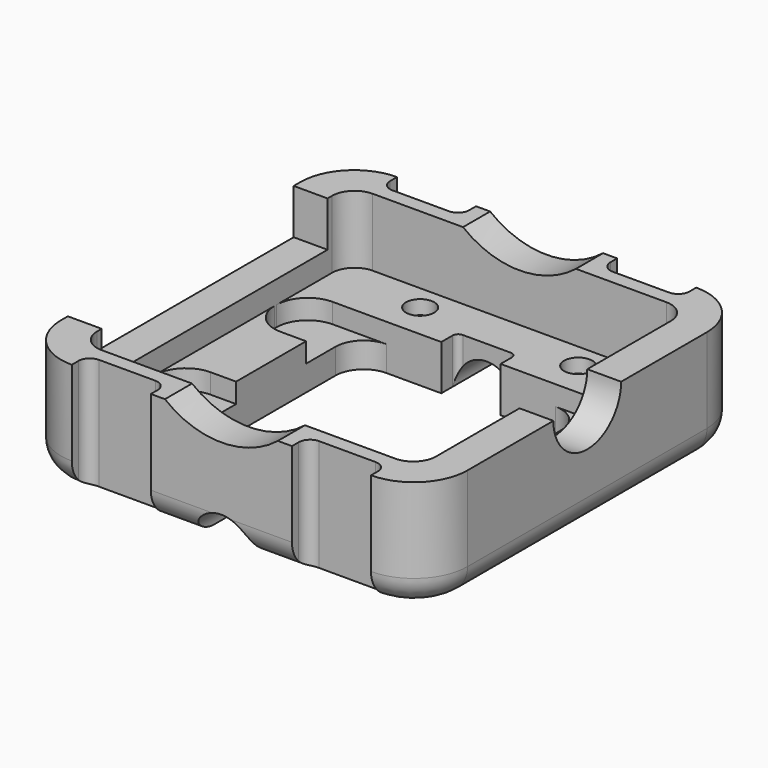
from build123d import *

# Parameters (mm, degrees)
F0_W           = 72
F0_H           = 72
F1_DEPTH       = 20
F2_W           = 60
F2_H           = 59.9999963053
F3_DEPTH       = 12
F4_W           = 40
F4_H           = 38.5
F5_DEPTH       = 8
F6_R           = 5.25
F7_DEPTH       = 72
F8_W           = 50
F8_H           = 16
F9_DEPTH       = 6.5
F10_R          = 7.5
F11_DEPTH      = 6.5
F12_W          = 10.5
F12_H          = 45.5
F13_DEPTH      = 12.001
F13_DEPTH_BACK = 8.001
F14_W          = 60
F14_H          = 11.5
F15_DEPTH      = 3.5
F16_W          = 14
F16_H          = 7
F17_DEPTH      = 20.001
F19_DEPTH      = 72.001
F21_T1_DEPTH   = 4.5
F21_T3_DEPTH   = 97
F21_T5_DEPTH   = 34.5
F21_T7_DEPTH   = 32.25
F21_T9_DEPTH   = 34.5
F21_T11_DEPTH  = 32.25
F22_R          = 2
F23_R          = 5.5
F24_R          = 4
F25_T4_DEPTH   = 8
F25_S5_R       = 5.25
F25_T6_DEPTH   = 6
F25_T10_DEPTH  = 8
F25_S11_R      = 5.25
F25_T12_DEPTH  = 6
F25_T16_DEPTH  = 8
F25_S17_R      = 5.25
F25_T18_DEPTH  = 6
F25_T22_DEPTH  = 8
F25_S23_R      = 5.25
F25_T24_DEPTH  = 6
F20_R          = 4.75
F20_R_2        = 2.5
F26_DEPTH      = 5.5
F27_DEPTH      = 20.0010001
F28_T1_DEPTH   = 43.7500000001
F28_T4_ANGLE   = 90
F28_T6_ANGLE   = 90
F28_T8_ANGLE   = 90
F28_T10_ANGLE  = 90


# Not quite as in the source:
# - a fillet or chamfer that OpenCascade refuses, or shapes differently, is made with other operations: its cross-section is extruded or revolved along the edge and cut away or added


with BuildPart() as f1:
    # F0 (on Top) → F1 (new body)
    with BuildSketch(Plane.XY):
        Rectangle(F0_W, F0_H)
    extrude(amount=F1_DEPTH)

    # F2 (on face) → F3 (cut)
    with BuildSketch(Plane.XY.offset(20)):
        Rectangle(F2_W, F2_H)
    extrude(amount=-F3_DEPTH, mode=Mode.SUBTRACT)

    # F4 (on face) → F5 (cut, through all)
    with BuildSketch(Plane.XY.offset(8)):
        Rectangle(F4_W, F4_H)
    extrude(amount=-F5_DEPTH, mode=Mode.SUBTRACT)

    # F6 (on face) → F7 (cut, through all)
    with BuildSketch(Plane.XZ.offset(36)):
        Circle(F6_R)
    extrude(amount=-F7_DEPTH, mode=Mode.SUBTRACT)

    # F8 (on face) → F9 (cut)
    with BuildSketch(Plane(origin=(-36, 0, 0), x_dir=(0, -1, 0), z_dir=(-1, 0, 0))):
        with Locations((0, 20)):
            Rectangle(F8_W, F8_H)
    extrude(amount=-F9_DEPTH, mode=Mode.SUBTRACT)

    # F10 (on face) → F11 (cut)
    with BuildSketch(Plane.YZ.offset(36)):
        with Locations((0, 20)):
            Circle(F10_R)
    extrude(amount=-F11_DEPTH, mode=Mode.SUBTRACT)

    # F12 (on face) → F13 (cut, two sides)
    with BuildSketch(Plane.XY.offset(8)) as f13_sk:
        Rectangle(F12_W, F12_H)
    extrude(amount=F13_DEPTH, mode=Mode.SUBTRACT)
    extrude(f13_sk.sketch, amount=-F13_DEPTH_BACK, mode=Mode.SUBTRACT)

    # F14 (on face) → F15 (cut)
    with BuildSketch(Plane.XY.offset(8)):
        with Locations((0, 13.5)):
            Rectangle(F14_W, F14_H)
        with Locations((0, -13.5)):
            Rectangle(F14_W, F14_H)
    extrude(amount=-F15_DEPTH, mode=Mode.SUBTRACT)

    # F16 (on face) → F17 (cut, through all)
    with BuildSketch(Plane.XY.offset(20)):
        with Locations((-19.5, 36)):
            Rectangle(F16_W, F16_H)
        with Locations((-19.5, -36)):
            Rectangle(F16_W, F16_H)
        with Locations((19.5, -36)):
            Rectangle(F16_W, F16_H)
        with Locations((19.5, 36)):
            Rectangle(F16_W, F16_H)
    extrude(amount=-F17_DEPTH, mode=Mode.SUBTRACT)

    # F18 (on face) → F19 (cut, through all)
    with BuildSketch(Plane(origin=(0, 36, 0), x_dir=(-1, 0, 0), z_dir=(0, 1, 0))):
        with BuildLine():
            Line((10, 20), (-10, 20))
            ThreePointArc((-10, 20), (0, 16.5), (10, 20))
        make_face()
    extrude(amount=-F19_DEPTH, mode=Mode.SUBTRACT)

    # F21: fillet of radius 5 on 14 edges, made by hand

    # F21_s2 → F21_t1 (join)
    with BuildSketch(Plane.XY):
        with BuildLine():
            ThreePointArc((20, 14.25), (18.5355339059, 17.7855339059), (15, 19.25))
            Line((15, 19.25), (20, 19.25))
            Line((20, 19.25), (20, 14.25))
        make_face()
        with BuildLine():
            ThreePointArc((-15, 19.25), (-18.5355339059, 17.7855339059), (-20, 14.25))
            Line((-20, 14.25), (-20, 19.25))
            Line((-20, 19.25), (-15, 19.25))
        make_face()
        with BuildLine():
            ThreePointArc((-20, -14.25), (-18.5355339059, -17.7855339059), (-15, -19.25))
            Line((-15, -19.25), (-20, -19.25))
            Line((-20, -19.25), (-20, -14.25))
        make_face()
        with BuildLine():
            ThreePointArc((15, -19.25), (18.5355339059, -17.7855339059), (20, -14.25))
            Line((20, -14.25), (20, -19.25))
            Line((20, -19.25), (15, -19.25))
        make_face()
    extrude(amount=F21_T1_DEPTH)

    # F21_s4 → F21_t3 (cut)
    with BuildSketch(Plane.XZ.offset(-48.5)):
        with BuildLine():
            ThreePointArc((36, 5), (34.5355339059, 1.4644660941), (31, 0))
            Line((31, 0), (36, 0))
            Line((36, 0), (36, 5))
        make_face()
        with BuildLine():
            ThreePointArc((-36, 5), (-34.5355339059, 1.4644660941), (-31, 0))
            Line((-31, 0), (-36, 0))
            Line((-36, 0), (-36, 5))
        make_face()
    extrude(amount=F21_T3_DEPTH, mode=Mode.SUBTRACT)

    # F21_s6 → F21_t5 (cut)
    with BuildSketch(Plane.YZ.offset(14)):
        with BuildLine():
            ThreePointArc((-36, 5), (-34.5355339059, 1.4644660941), (-31, 0))
            Line((-31, 0), (-36, 0))
            Line((-36, 0), (-36, 5))
        make_face()
        with BuildLine():
            ThreePointArc((36, 5), (34.5355339059, 1.4644660941), (31, 0))
            Line((31, 0), (36, 0))
            Line((36, 0), (36, 5))
        make_face()
    extrude(amount=F21_T5_DEPTH, mode=Mode.SUBTRACT)

    # F21_s8 → F21_t7 (cut)
    with BuildSketch(Plane.YZ.offset(-25)):
        with BuildLine():
            ThreePointArc((-36, 5), (-34.5355339059, 1.4644660941), (-31, 0))
            Line((-31, 0), (-36, 0))
            Line((-36, 0), (-36, 5))
        make_face()
        with BuildLine():
            ThreePointArc((36, 5), (34.5355339059, 1.4644660941), (31, 0))
            Line((31, 0), (36, 0))
            Line((36, 0), (36, 5))
        make_face()
    extrude(amount=F21_T7_DEPTH, mode=Mode.SUBTRACT)

    # F21_s10 → F21_t9 (cut)
    with BuildSketch(Plane.YZ.offset(-48.5)):
        with BuildLine():
            ThreePointArc((36, 5), (34.5355339059, 1.4644660941), (31, 0))
            Line((31, 0), (36, 0))
            Line((36, 0), (36, 5))
        make_face()
        with BuildLine():
            ThreePointArc((-36, 5), (-34.5355339059, 1.4644660941), (-31, 0))
            Line((-31, 0), (-36, 0))
            Line((-36, 0), (-36, 5))
        make_face()
    extrude(amount=F21_T9_DEPTH, mode=Mode.SUBTRACT)

    # F21_s12 → F21_t11 (cut)
    with BuildSketch(Plane.YZ.offset(-7.25)):
        with BuildLine():
            ThreePointArc((36, 5), (34.5355339059, 1.4644660941), (31, 0))
            Line((31, 0), (36, 0))
            Line((36, 0), (36, 5))
        make_face()
        with BuildLine():
            ThreePointArc((-36, 5), (-34.5355339059, 1.4644660941), (-31, 0))
            Line((-31, 0), (-36, 0))
            Line((-36, 0), (-36, 5))
        make_face()
    extrude(amount=F21_T11_DEPTH, mode=Mode.SUBTRACT)

    # F22
    f22_edges = [f1.edges().sort_by_distance(p)[0] for p in [
        (12.5, 32.5, 10.115152),
        (-26.5, 32.5, 10.115152),
        (-12.5, 32.5, 10.115152),
        (26.5, 32.5, 10.115152),
        (-26.5, -32.5, 10.115152),
        (12.5, -32.5, 10.115152),
        (-12.5, -32.5, 10.115152),
        (26.5, -32.5, 10.115152),
    ]]
    fillet(f22_edges, radius=F22_R)

    # F23
    f23_edges = [f1.edges().sort_by_distance(p)[0] for p in [
        (-30, 19.25, 6.25),
        (-30, 7.75, 6.25),
        (-30, -19.25, 6.25),
        (-30, -7.75, 6.25),
        (30, -19.25, 6.25),
        (30, -7.75, 6.25),
        (30, 19.25, 6.25),
        (30, 7.75, 6.25),
    ]]
    fillet(f23_edges, radius=F23_R)

    # F24
    f24_edges = [f1.edges().sort_by_distance(p)[0] for p in [
        (-30, -29.999998, 14),
        (-30, 29.999998, 14),
        (30, 29.999998, 14),
        (30, -29.999998, 14),
    ]]
    fillet(f24_edges, radius=F24_R)

    # F25: fillet of radius 1 on 4 edges, made by hand


with BuildPart() as f25_tool2:
    # F25_s3 → F25_t4 (new body)
    with BuildSketch(Plane.XY.offset(8)):
        with BuildLine():
            ThreePointArc((-4.25, 22.75), (-4.9571067812, 22.4571067812), (-5.25, 21.75))
            Line((-5.25, 21.75), (-5.25, 22.75))
            Line((-5.25, 22.75), (-4.25, 22.75))
        make_face()
    extrude(amount=-F25_T4_DEPTH)

    # F25_s5 → F25_t6 (cut, symmetric)
    with BuildSketch(Plane.XZ.offset(-22.2)):
        Circle(F25_S5_R)
    extrude(amount=F25_T6_DEPTH, both=True, mode=Mode.SUBTRACT)


with BuildPart() as f1_1:
    add(f1.part)

    # F25_t1: union F25_tool2
    add(f25_tool2.part)


with BuildPart() as f25_tool8:
    # F25_s9 → F25_t10 (new body)
    with BuildSketch(Plane.XY.offset(8)):
        with BuildLine():
            ThreePointArc((5.25, 21.75), (4.9571067812, 22.4571067812), (4.25, 22.75))
            Line((4.25, 22.75), (5.25, 22.75))
            Line((5.25, 22.75), (5.25, 21.75))
        make_face()
    extrude(amount=-F25_T10_DEPTH)

    # F25_s11 → F25_t12 (cut, symmetric)
    with BuildSketch(Plane.XZ.offset(-22.2)):
        Circle(F25_S11_R)
    extrude(amount=F25_T12_DEPTH, both=True, mode=Mode.SUBTRACT)


with BuildPart() as f1_2:
    add(f1_1.part)

    # F25_t7: union F25_tool8
    add(f25_tool8.part)


with BuildPart() as f25_tool14:
    # F25_s15 → F25_t16 (new body)
    with BuildSketch(Plane.XY):
        with BuildLine():
            ThreePointArc((5.25, -21.75), (4.9571067812, -22.4571067812), (4.25, -22.75))
            Line((4.25, -22.75), (5.25, -22.75))
            Line((5.25, -22.75), (5.25, -21.75))
        make_face()
    extrude(amount=F25_T16_DEPTH)

    # F25_s17 → F25_t18 (cut, symmetric)
    with BuildSketch(Plane.XZ.offset(22.2)):
        Circle(F25_S17_R)
    extrude(amount=F25_T18_DEPTH, both=True, mode=Mode.SUBTRACT)


with BuildPart() as f1_3:
    add(f1_2.part)

    # F25_t13: union F25_tool14
    add(f25_tool14.part)


with BuildPart() as f25_tool20:
    # F25_s21 → F25_t22 (new body)
    with BuildSketch(Plane.XY):
        with BuildLine():
            ThreePointArc((-4.25, -22.75), (-4.9571067812, -22.4571067812), (-5.25, -21.75))
            Line((-5.25, -21.75), (-5.25, -22.75))
            Line((-5.25, -22.75), (-4.25, -22.75))
        make_face()
    extrude(amount=F25_T22_DEPTH)

    # F25_s23 → F25_t24 (cut, symmetric)
    with BuildSketch(Plane.XZ.offset(22.2)):
        Circle(F25_S23_R)
    extrude(amount=F25_T24_DEPTH, both=True, mode=Mode.SUBTRACT)


with BuildPart() as f1_4:
    add(f1_3.part)

    # F25_t19: union F25_tool20
    add(f25_tool20.part)

    # F20 (on face) → F26 (cut)
    with BuildSketch(Plane(origin=(0, 0, 0), x_dir=(1, 0, 0), z_dir=(0, 0, -1))):
        with Locations((14, -25.5)):
            Circle(F20_R)
        with Locations((14, -25.5)):
            Circle(F20_R_2, mode=Mode.SUBTRACT)
        with Locations((-14, -25.5)):
            Circle(F20_R)
        with Locations((-14, -25.5)):
            Circle(F20_R_2, mode=Mode.SUBTRACT)
        with Locations((14, 25.5)):
            Circle(F20_R)
        with Locations((14, 25.5)):
            Circle(F20_R_2, mode=Mode.SUBTRACT)
        with Locations((-14, 25.5)):
            Circle(F20_R)
        with Locations((-14, 25.5)):
            Circle(F20_R_2, mode=Mode.SUBTRACT)
    extrude(amount=-F26_DEPTH, mode=Mode.SUBTRACT)

    # F27 (cut, through all): faces of the model
    f27_faces = [f1_4.faces().sort_by_distance(p)[0] for p in [
        (14, 25.5, 0),
        (-14, 25.5, 0),
        (-14, -25.5, 0),
        (14, -25.5, 0),
    ]]
    extrude(f27_faces, amount=-F27_DEPTH, mode=Mode.SUBTRACT)

    # F28: fillet of radius 9.5 on 4 edges, made by hand

    # F28_s2 → F28_t1 (cut)
    with BuildSketch(Plane.XY):
        with BuildLine():
            ThreePointArc((36, -26.5), (33.2175144213, -33.2175144213), (26.5, -36))
            Line((26.5, -36), (36, -36))
            Line((36, -36), (36, -26.5))
        make_face()
        with BuildLine():
            ThreePointArc((-36, -26.5), (-33.2175144213, -33.2175144213), (-26.5, -36))
            Line((-26.5, -36), (-36, -36))
            Line((-36, -36), (-36, -26.5))
        make_face()
        with BuildLine():
            ThreePointArc((-36, 26.5), (-33.2175144213, 33.2175144213), (-26.5, 36))
            Line((-26.5, 36), (-36, 36))
            Line((-36, 36), (-36, 26.5))
        make_face()
        with BuildLine():
            ThreePointArc((36, 26.5), (33.2175144213, 33.2175144213), (26.5, 36))
            Line((26.5, 36), (36, 36))
            Line((36, 36), (36, 26.5))
        make_face()
    extrude(amount=F28_T1_DEPTH, mode=Mode.SUBTRACT)

    # F28_s3 → F28_t4 (revolve, cut)
    with BuildSketch(Plane.YZ.offset(26.5)):
        with BuildLine():
            ThreePointArc((30.9999999999, 0), (34.5355339059, 1.4644660941), (36, 5.0000000001))
            Line((36, 5.0000000001), (36, 0))
            Line((36, 0), (30.9999999999, 0))
        make_face()
    revolve(axis=Axis((26.5, 26.5, 0), (0, 0, -1)), revolution_arc=F28_T4_ANGLE, mode=Mode.SUBTRACT)

    # F28_s5 → F28_t6 (revolve, cut)
    with BuildSketch(Plane.XZ.offset(-26.5)):
        with BuildLine():
            ThreePointArc((-30.9999999999, 0), (-34.5355339059, 1.4644660941), (-36, 5.0000000001))
            Line((-36, 5.0000000001), (-36, 0))
            Line((-36, 0), (-30.9999999999, 0))
        make_face()
    revolve(axis=Axis((-26.5, 26.5, 0), (0, 0, -1)), revolution_arc=F28_T6_ANGLE, mode=Mode.SUBTRACT)

    # F28_s7 → F28_t8 (revolve, cut)
    with BuildSketch(Plane.YZ.offset(-26.5)):
        with BuildLine():
            ThreePointArc((-30.9999999999, 0), (-34.5355339059, 1.4644660941), (-36, 5.0000000001))
            Line((-36, 5.0000000001), (-36, 0))
            Line((-36, 0), (-30.9999999999, 0))
        make_face()
    revolve(axis=Axis((-26.5, -26.5, 0), (0, 0, -1)), revolution_arc=F28_T8_ANGLE, mode=Mode.SUBTRACT)

    # F28_s9 → F28_t10 (revolve, cut)
    with BuildSketch(Plane.XZ.offset(26.5)):
        with BuildLine():
            ThreePointArc((30.9999999999, 0), (34.5355339059, 1.4644660941), (36, 5.0000000001))
            Line((36, 5.0000000001), (36, 0))
            Line((36, 0), (30.9999999999, 0))
        make_face()
    revolve(axis=Axis((26.5, -26.5, 0), (0, 0, -1)), revolution_arc=F28_T10_ANGLE, mode=Mode.SUBTRACT)


solid = f1_4.part
